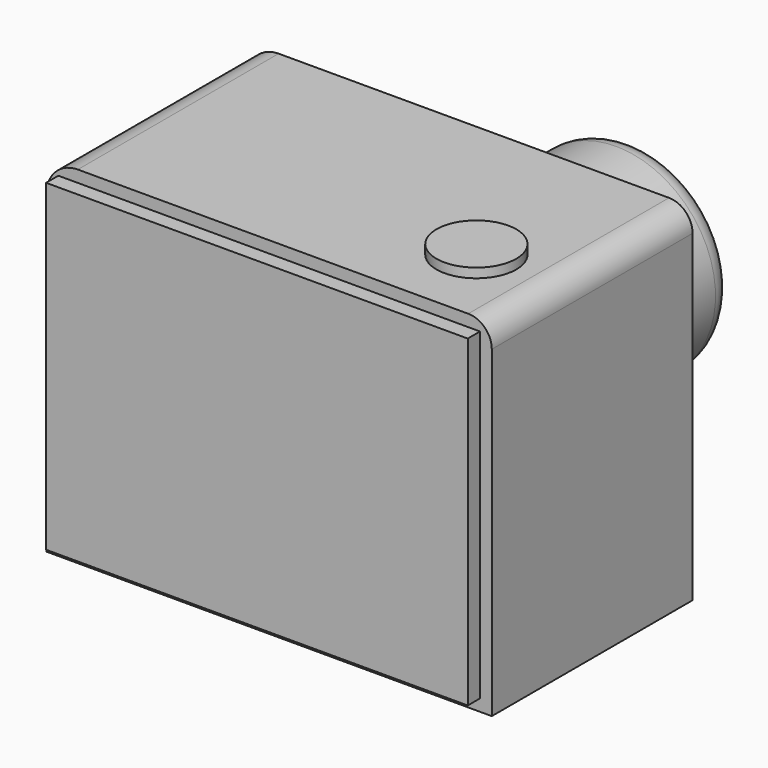
from build123d import *

# Parameters (mm, degrees)
F0_W         = 95.9731452167
F0_H         = 74.7115183622
F1_DEPTH     = 54.102
F2_T         = -2.54
F3_R         = 21.4425238222
F4_DEPTH     = 34.798
F5_R         = 6.7453126933
F6_R         = 5.08
F7_R         = 5.08
F8_TEXT_SIZE = 15.5540726458
F9_DEPTH     = 5.588
F10_R        = 8.6096383386
F11_DEPTH    = 2.032
F12_W        = 90.8931452167
F12_H        = 69.6315183622
F13_DEPTH    = 54.864


# Not quite as in the source:
# - Text() gives the source's letters only with a copy of the font that has no kerning and outlines rounded to 1/6400 em; it was checked with that copy


with BuildPart() as f1:
    # F0 (on Front) → F1 (new body)
    with BuildSketch(Plane.XZ):
        with Locations((-16.4476949722, 11.8692172691)):
            Rectangle(F0_W, F0_H)
    extrude(amount=F1_DEPTH)

    # F2
    f2_openings = [f1.faces().sort_by_distance(p)[0] for p in [
        (-16.447695, -54.102, 11.869217),
    ]]
    offset(amount=F2_T, openings=f2_openings)

    # F3 (on face) → F4 (join)
    with BuildSketch(Plane(origin=(0, 0, 0), x_dir=(-1, 0, 0), z_dir=(0, 1, 0))):
        with Locations((8.7343109772, 14.0373446047)):
            Circle(F3_R)
    extrude(amount=F4_DEPTH)

    # F5
    f5_edges = [f1.edges().sort_by_distance(p)[0] for p in [
        (-64.434268, -27.051, 49.224976),
    ]]
    fillet(f5_edges, radius=F5_R)

    # F6
    f6_edges = [f1.edges().sort_by_distance(p)[0] for p in [
        (31.538878, -27.051, 49.224976),
    ]]
    fillet(f6_edges, radius=F6_R)

    # F7
    f7_edges = [f1.edges().sort_by_distance(p)[0] for p in [
        (12.708213, 34.798, 14.037345),
    ]]
    fillet(f7_edges, radius=F7_R)

    # F8 (on face) → F9 (join)
    with BuildSketch(Plane(origin=(0, 0, 0), x_dir=(-1, 0, 0), z_dir=(0, 1, 0))):
        with Locations((21.5052496642, -21.4725770056)):
            Text('SONY', F8_TEXT_SIZE, font='Open Sans', text_align=(TextAlign.LEFT, TextAlign.BOTTOM))
    extrude(amount=F9_DEPTH)

    # F10 (on face) → F11 (join)
    with BuildSketch(Plane.XY.offset(49.2249764502)):
        with Locations((14.0883233398, -36.4437922835)):
            Circle(F10_R)
    extrude(amount=F11_DEPTH)

    # F12 (on face) → F13 (join)
    with BuildSketch(Plane.XZ.offset(2.54)):
        with Locations((-16.4476949722, 11.8692172691)):
            Rectangle(F12_W, F12_H)
    extrude(amount=F13_DEPTH)


solid = f1.part
